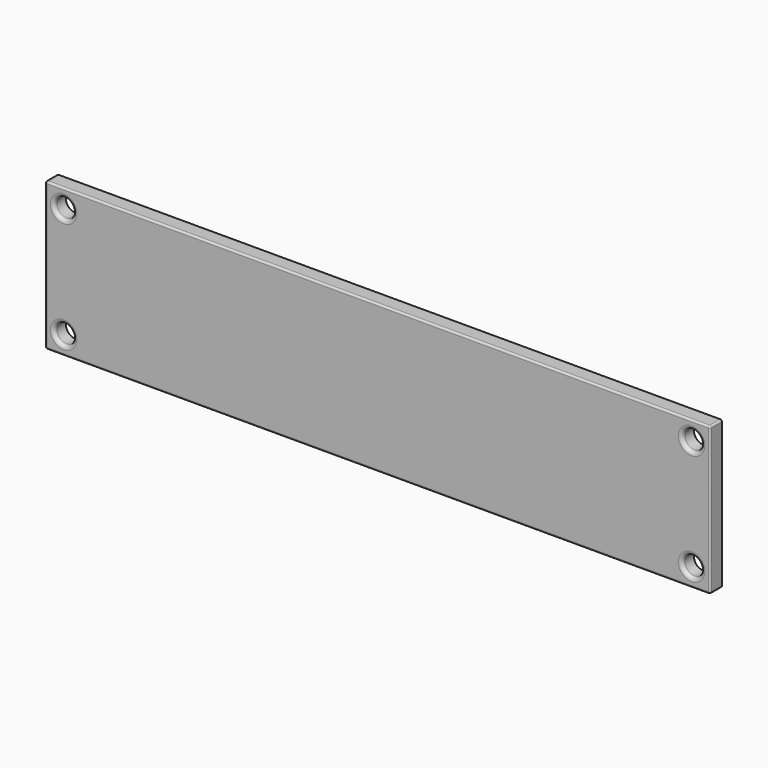
from build123d import *

# Parameters (mm, degrees)
F0_W         = 180
F0_H         = 40
F0_R         = 2.5751263091
F1_DEPTH     = 4
F2_R         = 1
F3_R         = 0.5
F4_TEXT_SIZE = 22.6015303119
F5_DEPTH     = 1


# Not quite as in the source:
# - a feature names something its author has since deleted; it is built from what else it names
# - Text() gives the source's letters only with a copy of the font that has no kerning and outlines rounded to 1/6400 em; it was checked with that copy


with BuildPart() as f1:
    # F0 (on Front) → F1 (new body)
    with BuildSketch(Plane.XZ):
        Rectangle(F0_W, F0_H)
        with Locations((-85, -15)):
            Circle(F0_R, mode=Mode.SUBTRACT)
        with Locations((85, -15)):
            Circle(F0_R, mode=Mode.SUBTRACT)
        with Locations((-85, 15)):
            Circle(F0_R, mode=Mode.SUBTRACT)
        with Locations((85, 15)):
            Circle(F0_R, mode=Mode.SUBTRACT)
    extrude(amount=F1_DEPTH)

    # F2
    f2_edges = [f1.edges().sort_by_distance(p)[0] for p in [
        (-87.575126, -4, 15),
        (-87.575126, -4, -15),
        (82.424874, -4, 15),
        (82.424874, -4, -15),
    ]]
    fillet(f2_edges, radius=F2_R)

    # F3
    f3_edges = [f1.edges().sort_by_distance(p)[0] for p in [
        (0, -4, 20),
        (-90, -4, 0),
        (0, -4, -20),
        (90, -4, 0),
        (-90, -2, 20),
        (-90, -2, -20),
        (90, -2, 20),
        (90, -2, -20),
    ]]
    fillet(f3_edges, radius=F3_R)

    # F4 (on face) → F5 (join)
    with BuildSketch(Plane(origin=(0, 0, 0), x_dir=(-1, 0, 0), z_dir=(0, 1, 0))):
        with Locations((-67.0919371769, -8.4678279565)):
            Text('Sierra', F4_TEXT_SIZE, font='Open Sans', text_align=(TextAlign.LEFT, TextAlign.BOTTOM))
    extrude(amount=F5_DEPTH)

    # F6: F1 across plane


with BuildPart() as f1_1:
    add(f1.part)
    add(f1.part.mirror(Plane.YZ))


solid = f1_1.part
